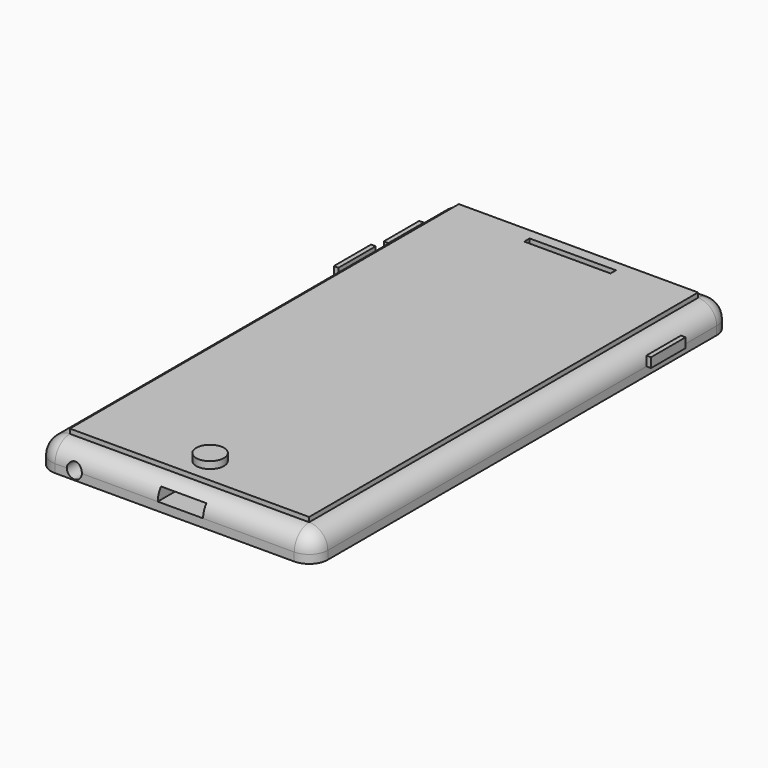
from build123d import *

# Parameters (mm, degrees)
F0_W      = 75.4051078111
F0_H      = 142.7516564727
F1_DEPTH  = 7.366
F2_F1_R   = 5.08
F2_F2_R   = 5.08
F2_F3_R   = 5.08
F2_F4_R   = 5.08
F3_W      = 12.3756472021
F3_H      = 3.1823093913
F4_DEPTH  = 6.35
F5_R      = 2.046755254
F6_DEPTH  = 6.35
F7_W      = 65.2451078111
F7_H      = 132.5916564727
F8_DEPTH  = 1.27
F9_W      = 11.800032109
F9_H      = 2.6066980235
F10_DEPTH = 1.27
F11_R     = 3.7854916829
F12_DEPTH = 1.905
F13_W     = 23.5232524574
F13_H     = 1.857098192
F14_DEPTH = 6.35
F15_W     = 12.0711438358
F15_H     = 2.5115047491
F16_DEPTH = 1.27
F17_W     = 12.7
F17_H     = 3.5076188103
F18_DEPTH = 1.27
F20_DEPTH = 1.27


with BuildPart() as f1:
    # F0 (on Top) → F1 (new body)
    with BuildSketch(Plane.XY):
        with Locations((-26.1903246865, -3.4536682069)):
            Rectangle(F0_W, F0_H)
    extrude(amount=F1_DEPTH)

    # F2: fillet of radius 5.08 on 8 edges, made by hand

    # F2_f1
    f2_f1_edges = [f1.edges().sort_by_distance(p)[0] for p in [
        (11.5122292191, 67.9221600294, 3.683),
    ]]
    fillet(f2_f1_edges, radius=F2_F1_R)

    # F2_f2
    f2_f2_edges = [f1.edges().sort_by_distance(p)[0] for p in [
        (-63.892878592, 67.9221600294, 3.683),
    ]]
    fillet(f2_f2_edges, radius=F2_F2_R)

    # F2_f3
    f2_f3_edges = [f1.edges().sort_by_distance(p)[0] for p in [
        (-26.1903246865, 67.9221600294, 7.366),
    ]]
    fillet(f2_f3_edges, radius=F2_F3_R)

    # F2_f4
    f2_f4_edges = [f1.edges().sort_by_distance(p)[0] for p in [
        (-63.892878592, -74.8294964433, 1.143),
    ]]
    fillet(f2_f4_edges, radius=F2_F4_R)

    # F3 (on face) → F4 (cut)
    with BuildSketch(Plane.XZ.offset(74.8294964433)):
        with Locations((-24.6073929593, 3.8771546956)):
            Rectangle(F3_W, F3_H)
    extrude(amount=-F4_DEPTH, mode=Mode.SUBTRACT)

    # F5 (on face) → F6 (cut)
    with BuildSketch(Plane.XZ.offset(74.8294964433)):
        with Locations((-53.5318702459, 2.286)):
            Circle(F5_R)
    extrude(amount=-F6_DEPTH, mode=Mode.SUBTRACT)


with BuildPart() as f8:
    # F7 (on face) → F8 (new body)
    with BuildSketch(Plane.XY.offset(7.366)):
        with Locations((-26.1903246865, -3.4536682069)):
            Rectangle(F7_W, F7_H)
    extrude(amount=F8_DEPTH)

    # F13 (on face) → F14 (cut)
    with BuildSketch(Plane.XY.offset(8.636)):
        with Locations((-25.3803487867, 58.9628834277)):
            Rectangle(F13_W, F13_H)
    extrude(amount=-F14_DEPTH, mode=Mode.SUBTRACT)


with BuildPart() as f10:
    # F9 (on face) → F10 (new body)
    with BuildSketch(Plane.YZ.offset(11.5122292191)):
        with Locations((44.7537954897, 3.5893490117)):
            Rectangle(F9_W, F9_H)
    extrude(amount=F10_DEPTH)


with BuildPart() as f12:
    # F11 (on face) → F12 (new body)
    with BuildSketch(Plane.XY.offset(8.636)):
        with Locations((-26.1903246865, -62.7416521311)):
            Circle(F11_R)
    extrude(amount=F12_DEPTH)


with BuildPart() as f16:
    # F15 (on face) → F16 (new body)
    with BuildSketch(Plane(origin=(-63.892878592, 0, 0), x_dir=(0, -1, 0), z_dir=(-1, 0, 0))):
        with Locations((-51.2249711901, 3.5417523746)):
            Rectangle(F15_W, F15_H)
    extrude(amount=F16_DEPTH)


with BuildPart() as f18:
    # F17 (on face) → F18 (new body)
    with BuildSketch(Plane(origin=(-63.892878592, 0, 0), x_dir=(0, -1, 0), z_dir=(-1, 0, 0))):
        with Locations((-34.5061713994, 4.0398094052)):
            Rectangle(F17_W, F17_H)
    extrude(amount=F18_DEPTH)


with BuildPart() as f20:
    # F19 (on face) → F20 (new body)
    with BuildSketch(Plane(origin=(0, 0, 0), x_dir=(1, 0, 0), z_dir=(0, 0, -1))):
        with BuildLine():
            add(Edge.make_bspline(
                [(-26.9279293716, -37.296731025), (-26.1590478095, -37.8796180067), (-27.2405076799, -41.610190349), (-33.6150642057, -44.8689171286), (-32.8227501646, -38.2996334195), (-27.8316461583, -36.6116258331), (-26.9279293716, -37.296731025)],
                knots=[0, 0, 0, 0, 0.2291805231, 0.4943005153, 0.7306291422, 1, 1, 1, 1], degree=3))
        make_face()
    extrude(amount=F20_DEPTH)


with BuildPart() as f20b:
    # F19 (on face) → F20, piece 2 (new body)
    with BuildSketch(Plane(origin=(0, 0, 0), x_dir=(1, 0, 0), z_dir=(0, 0, -1))):
        with BuildLine():
            add(Edge.make_bspline(
                [(-18.5709875077, -34.8206013441), (-16.9933307569, -34.4069620178), (-14.1792039609, -33.0899210778), (-13.7777924329, -27.883110785), (-14.272988719, -21.6169154673), (-16.351813669, -16.762216435), (-21.0363385209, -9.9297464764), (-26.8947206756, -14.9211673759), (-32.2389811264, -11.130286541), (-36.3725185757, -14.0623640639), (-39.5224923345, -18.8545713408), (-37.2114139136, -21.0298104682), (-34.5153706863, -27.1103805858), (-36.2968935413, -29.969179565), (-39.0716980584, -31.7151857926), (-37.5791604466, -35.9829722305), (-31.7963960221, -34.5523022934), (-29.4355823464, -34.9774247098), (-26.8124785552, -32.318446701), (-23.9298221224, -35.599274808), (-20.3161966458, -35.2781705408), (-18.5709875077, -34.8206013441)],
                knots=[0, 0, 0, 0, 0.0520581477, 0.10668462, 0.1693019503, 0.2291883895, 0.2935167278, 0.3538845551, 0.4122524688, 0.4659202448, 0.522004706, 0.5637754073, 0.6266239453, 0.6704560449, 0.7128646393, 0.7566967388, 0.814283655, 0.8539413629, 0.8957120516, 0.9424131041, 1, 1, 1, 1], degree=3))
        make_face()
    extrude(amount=F20_DEPTH)


solid = Compound([f1.part, f8.part, f10.part, f12.part, f16.part, f18.part, f20.part, f20b.part])
